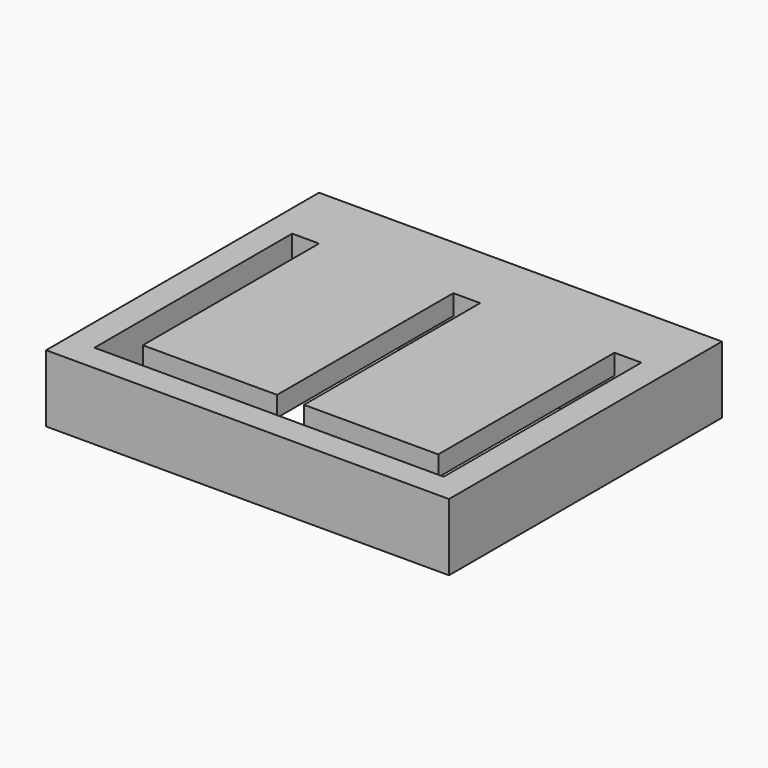
from build123d import *

# Parameters (mm, degrees)
F0_W         = 30
F0_H         = 25.4
F1_DEPTH     = 5
F2_W         = 22
F2_H         = 16.4
F3_DEPTH     = 3.5
F4_R         = 1.5
F5_DEPTH     = 2
F6_TEXT_SIZE = 4.8611111111
F7_DEPTH     = 1


# Not quite as in the source:
# - Text() gives the source's letters only with a copy of the font that has no kerning and outlines rounded to 1/6400 em; it was checked with that copy


with BuildPart() as f1:
    # F0 (on Top) → F1 (new body)
    with BuildSketch(Plane.XY):
        Rectangle(F0_W, F0_H)
        Polygon((-13, 7.7), (-11, 7.7), (-11, -8.7), (-1, -8.7), (-1, 7.7), (1, 7.7), (1, -8.7), (11, -8.7), (11, 7.7), (13, 7.7), (13, -10.7), (-13, -10.7), align=None, mode=Mode.SUBTRACT)
    extrude(amount=F1_DEPTH)

    # F2 (on face) → F3 (cut)
    with BuildSketch(Plane(origin=(0, 0, 0), x_dir=(1, 0, 0), z_dir=(0, 0, -1))):
        with Locations((0, 0.5)):
            Rectangle(F2_W, F2_H)
    extrude(amount=-F3_DEPTH, mode=Mode.SUBTRACT)

    # F4 (on face) → F5 (join)
    with BuildSketch(Plane(origin=(0, 0, 3.5), x_dir=(1, 0, 0), z_dir=(0, 0, -1))):
        with Locations((6, 6.7)):
            Circle(F4_R)
        with Locations((-6, 6.7)):
            Circle(F4_R)
    extrude(amount=F5_DEPTH)

    # F6 (on face) → F7 (cut)
    with BuildSketch(Plane(origin=(0, 0, 0), x_dir=(1, 0, 0), z_dir=(0, 0, -1))):
        with Locations((-4.4881727431, -11.95)):
            Text('ABS', F6_TEXT_SIZE, font='Open Sans', text_align=(TextAlign.LEFT, TextAlign.BOTTOM))
    extrude(amount=-F7_DEPTH, mode=Mode.SUBTRACT)


solid = f1.part
